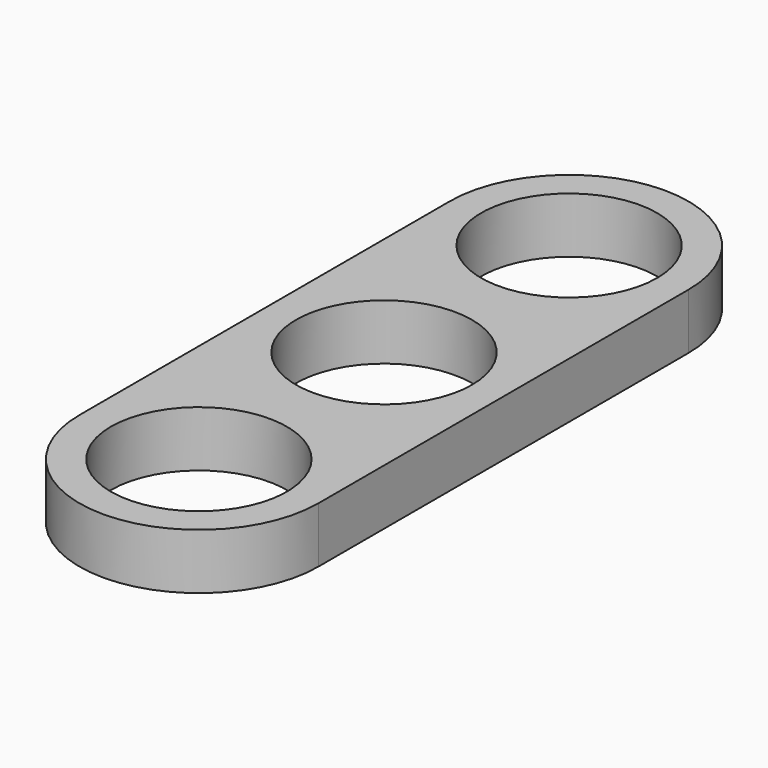
from build123d import *

# Parameters (mm, degrees)
F0_R     = 11.05
F1_DEPTH = 7
F2_DEPTH = 7
F3_COUNT = 2


with BuildPart() as f1:
    # F0 (on Top) → F1 (new body)
    with BuildSketch(Plane.XY):
        with BuildLine():
            ThreePointArc((-15, 0), (0, -15), (15, 0))
            ThreePointArc((15, 0), (0, 15), (-15, 0))
        make_face()
        Circle(F0_R, mode=Mode.SUBTRACT)
    extrude(amount=F1_DEPTH)



with BuildPart() as f2:
    # F0 (on Top) → F2 (new body, through all)
    with BuildSketch(Plane.XY):
        with BuildLine():
            ThreePointArc((-15, 0), (0, 15), (15, 0))
            Line((15, 0), (15, 29.05))
            ThreePointArc((15, 29.05), (0, 44.05), (-15, 29.05))
            Line((-15, 29.05), (-15, 0))
        make_face()
        with Locations((0, 29.05)):
            Circle(F0_R, mode=Mode.SUBTRACT)
    extrude(amount=F2_DEPTH)


with BuildPart() as f1_1:
    add(f1.part)

    add(f2.part)  # F3 merges F2
    # F3: F2 ×2 about axis
    f3_axis = Axis((0, 0, 0), (0, 0, 1))
    for i in range(1, F3_COUNT):
        add(f2.part.rotate(f3_axis, i * 360 / F3_COUNT))


solid = f1_1.part
